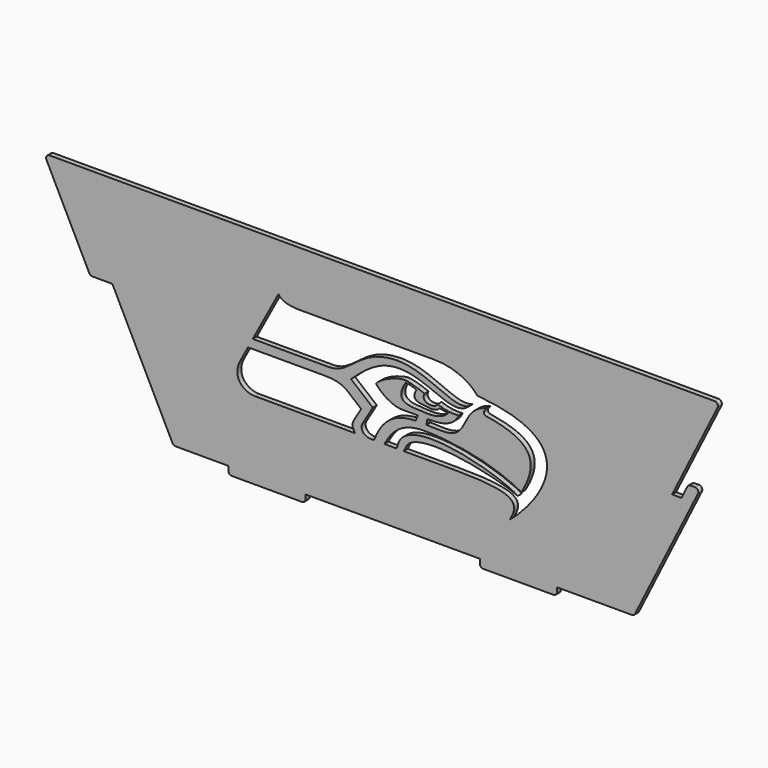
from build123d import *

# Parameters (mm, degrees)
F1_DEPTH = 4.7625
F3_DEPTH = 4.7635


with BuildPart() as f1:
    # F0 (on Front) → F1 (new body)
    with BuildSketch(Plane.XZ):
        with BuildLine():
            Line((304.8471037094, 203.7780743591), (-309.9778465366, 203.7780743591))
            Line((-309.9778465366, 203.7780743591), (-325.0692571728, 203.7780743591))
            ThreePointArc((-325.0692571728, 203.7780743591), (-327.7691254871, 202.2738035667), (-327.9106737709, 199.1863963025))
            Line((-327.9106737709, 199.1863963025), (-287.3259657756, 117.7860651637))
            ThreePointArc((-287.3259657756, 117.7860651637), (-286.1552783851, 116.502874906), (-284.4845491775, 116.0277432204))
            Line((-284.4845491775, 116.0277432204), (-265.4942987936, 116.0277432204))
            Line((-265.4942987936, 116.0277432204), (-208.521666982, 1.7583219434))
            ThreePointArc((-208.521666982, 1.7583219434), (-207.3509795915, 0.4751316856), (-205.6802503839, 0))
            Line((-205.6802503839, 0), (-155.575, 0))
            Line((-155.575, 0), (-155.575, -4.191))
            ThreePointArc((-155.575, -4.191), (-154.6450640303, -6.4360640303), (-152.4, -7.366))
            Line((-152.4, -7.366), (-85.725, -7.366))
            ThreePointArc((-85.725, -7.366), (-83.4799359697, -6.4360640303), (-82.55, -4.191))
            Line((-82.55, -4.191), (-82.55, 0))
            Line((-82.55, 0), (82.55, 0))
            Line((82.55, 0), (82.55, -4.191))
            ThreePointArc((82.55, -4.191), (83.4799359697, -6.4360640303), (85.725, -7.366))
            Line((85.725, -7.366), (152.4, -7.366))
            ThreePointArc((152.4, -7.366), (154.6450640303, -6.4360640303), (155.575, -4.191))
            Line((155.575, -4.191), (155.575, 0))
            Line((155.575, 0), (226.6352503839, 0))
            ThreePointArc((226.6352503839, 0), (228.3059795915, 0.4751316856), (229.476666982, 1.7583219434))
            Line((229.476666982, 1.7583219434), (289.1203551674, 121.3850534994))
            ThreePointArc((289.1203551674, 121.3850534994), (288.9788068837, 124.4724607637), (286.2789385693, 125.9767315561))
            Line((286.2789385693, 125.9767315561), (282.0216431033, 125.9767315561))
            ThreePointArc((282.0216431033, 125.9767315561), (280.3509138957, 125.5015998704), (279.1802265053, 124.2184096127))
            Line((279.1802265053, 124.2184096127), (273.5135142788, 112.8527432204))
            Line((273.5135142788, 112.8527432204), (264.6441487246, 112.8527432204))
            Line((264.6441487246, 112.8527432204), (307.6885203074, 199.1863963025))
            ThreePointArc((307.6885203074, 199.1863963025), (307.5469720237, 202.2738035667), (304.8471037094, 203.7780743591))
        make_face()
    extrude(amount=-F1_DEPTH)

    # F2 (on face) → F3 (cut, through all)
    with BuildSketch(Plane.XZ):
        with BuildLine():
            add(Edge.make_bspline(
                [(-108.0855709555, 158.8200743591), (-104.9123463275, 152.4905528223), (-92.8046389769, 151.9620743591), (-89.1326591372, 151.9620743591)],
                knots=[0, 0, 0, 0, 20.1555210895, 20.1555210895, 20.1555210895, 20.1555210895], degree=3))
            Line((-108.0855709555, 158.8200743591), (-132.5024012116, 113.3540743591))
            Line((-132.5024012116, 113.3540743591), (-60.2126787959, 113.3540743591))
            add(Edge.make_bspline(
                [(-60.2126787959, 113.3540743591), (-39.1802881973, 113.3540743591), (-32.2392965277, 139.1934752464), (3.4948316792, 139.8413479328)],
                knots=[0, 0, 0, 0, 68.994366091, 68.994366091, 68.994366091, 68.994366091], degree=3))
            add(Edge.make_bspline(
                [(3.4948316792, 139.8413479328), (33.620741922, 140.3875415964), (57.5292114558, 116.1221712828), (72.603527868, 124.0668594837)],
                knots=[0, 0, 0, 0, 70.8861507965, 70.8861507965, 70.8861507965, 70.8861507965], degree=3))
            add(Edge.make_bspline(
                [(72.603527868, 124.0668594837), (57.3887829127, 108.9602857828), (35.1666625979, 133.7167322636), (6.5191294456, 133.8571608067)],
                knots=[0, 0, 0, 0, 66.8056712775, 66.8056712775, 66.8056712775, 66.8056712775], degree=3))
            add(Edge.make_bspline(
                [(6.5191294456, 133.8571608067), (-10.7343354961, 133.9417362894), (-23.3095789241, 125.1955926418), (-39.4589209842, 110.169686377)],
                knots=[0, 0, 0, 0, 51.721152019, 51.721152019, 51.721152019, 51.721152019], degree=3))
            Line((-39.4589209842, 110.169686377), (-18.8014073711, 93.0641664272))
            Line((-18.8014073711, 93.0641664272), (-28.5283795675, 76.7167973694))
            add(Edge.make_bspline(
                [(-28.5283795675, 76.7167973694), (-31.1035539324, 72.3889011976), (-28.2070931256, 66.294), (-19.8544518154, 66.294)],
                knots=[0, 0, 0, 0, 13.5599309604, 13.5599309604, 13.5599309604, 13.5599309604], degree=3))
            Line((-19.8544518154, 66.294), (-17.6944385452, 66.294))
            Line((-17.6944385452, 66.294), (-15.5441686511, 71.12))
            add(Edge.make_bspline(
                [(21.8052406029, 95.3664587708), (7.467065883, 94.8295469973), (-6.8637521331, 90.6020614063), (-15.5441686511, 71.12)],
                knots=[43.7475476307, 43.7475476307, 43.7475476307, 43.7475476307, 82.7254389845, 82.7254389845, 82.7254389845, 82.7254389845], degree=3))
            Line((21.8052406029, 95.3664587708), (23.9405263848, 100.4171879244))
            Line((23.9405263848, 100.4171879244), (9.3578106412, 100.4171879244))
            add(Edge.make_bspline(
                [(-15.7739197216, 113.8468384743), (-9.2178139216, 106.1980500817), (0.431748606, 100.4171879244), (9.3578106412, 100.4171879244)],
                knots=[0, 0, 0, 0, 28.4949010337, 28.4949010337, 28.4949010337, 28.4949010337], degree=3))
            add(Edge.make_bspline(
                [(13.4090365761, 125.7664517022), (6.1268161537, 127.0878911018), (-12.3137527457, 119.4923743606), (-15.7739197216, 113.8468384743)],
                knots=[0, 0, 0, 0, 31.5233582883, 31.5233582883, 31.5233582883, 31.5233582883], degree=3))
            add(Edge.make_bspline(
                [(13.4090365761, 125.7664517022), (17.0461437806, 125.1064583922), (20.456541102, 124.1535529113), (23.7161297893, 123.0590063051)],
                knots=[0, 0, 0, 0, 9.7414046888, 9.7414046888, 9.7414046888, 9.7414046888], degree=3))
            add(Edge.make_bspline(
                [(23.7161297893, 123.0590063051), (25.9461937878, 122.3101667382), (28.1056690745, 121.4950294779), (30.2188615937, 120.6620362251)],
                knots=[9.7414046888, 9.7414046888, 9.7414046888, 9.7414046888, 16.4060357128, 16.4060357128, 16.4060357128, 16.4060357128], degree=3))
            add(Edge.make_bspline(
                [(30.2188615937, 120.6620362251), (34.4613134246, 118.989716397), (38.5172239418, 117.2454285237), (42.5832667432, 115.8211427133)],
                knots=[16.4060357128, 16.4060357128, 16.4060357128, 16.4060357128, 29.785969549, 29.785969549, 29.785969549, 29.785969549], degree=3))
            add(Edge.make_bspline(
                [(42.5832667432, 115.8211427133), (43.6102126796, 115.4614159232), (44.6378049525, 115.1221020021), (45.6692122023, 114.8095160445)],
                knots=[29.785969549, 29.785969549, 29.785969549, 29.785969549, 33.1652917436, 33.1652917436, 33.1652917436, 33.1652917436], degree=3))
            add(Edge.make_bspline(
                [(45.6692122023, 114.8095160445), (48.3287241294, 114.0035045657), (51.0136010899, 113.3752020751), (53.778166648, 113.0328753327)],
                knots=[33.1652917436, 33.1652917436, 33.1652917436, 33.1652917436, 41.8789668545, 41.8789668545, 41.8789668545, 41.8789668545], degree=3))
            add(Edge.make_bspline(
                [(53.778166648, 113.0328753327), (56.6101394852, 112.6822017765), (59.5257343252, 112.6316196452), (62.5833460553, 112.9975098393)],
                knots=[41.8789668545, 41.8789668545, 41.8789668545, 41.8789668545, 50.8051039667, 50.8051039667, 50.8051039667, 50.8051039667], degree=3))
            add(Edge.make_bspline(
                [(62.5833460553, 112.9975098393), (57.5499871238, 101.6970577857), (44.895685374, 100.4171879244), (35.6732808673, 100.4171879244)],
                knots=[0, 0, 0, 0, 29.7054895248, 29.7054895248, 29.7054895248, 29.7054895248], degree=3))
            Line((35.6732808673, 100.4171879244), (32.955760204, 100.4171879244))
            Line((32.955760204, 100.4171879244), (31.936584741, 95.2798231627))
            add(Edge.make_bspline(
                [(62.1327087283, 99.5770022273), (55.7191114325, 93.5406797473), (44.3494086047, 94.7811794741), (31.936584741, 95.2798231627)],
                knots=[0, 0, 0, 0, 34.4997978654, 34.4997978654, 34.4997978654, 34.4997978654], degree=3))
            add(Edge.make_bspline(
                [(89.5263329148, 127.8310716152), (69.5112124085, 122.403241694), (71.6838326954, 108.5662888403), (62.1327087283, 99.5770022273)],
                knots=[0, 0, 0, 0, 39.3535650615, 39.3535650615, 39.3535650615, 39.3535650615], degree=3))
            add(Edge.make_bspline(
                [(88.5086134076, 120.820119977), (86.8319925342, 121.0770893363), (84.3538343906, 123.8052621484), (89.5263329148, 127.8310716152)],
                knots=[0, 0, 0, 0, 7.0844333485, 7.0844333485, 7.0844333485, 7.0844333485], degree=3))
            add(Edge.make_bspline(
                [(121.9802498817, 68.2379975915), (138.7160643935, 97.1864387393), (133.5143968463, 113.9222532511), (88.5086134076, 120.820119977)],
                knots=[0, 0, 0, 0, 62.3316135105, 62.3316135105, 62.3316135105, 62.3316135105], degree=3))
            add(Edge.make_bspline(
                [(47.0553375781, 88.7687131763), (73.0637013912, 86.6201967001), (100.202858448, 80.1746398211), (121.9802498817, 68.2379975915)],
                knots=[0, 0, 0, 0, 77.6868892809, 77.6868892809, 77.6868892809, 77.6868892809], degree=3))
            add(Edge.make_bspline(
                [(-4.9613900483, 71.12), (7.5904717669, 91.8218642473), (26.8748909697, 90.4357931335), (47.0553375781, 88.7687131763)],
                knots=[0, 0, 0, 0, 54.9292001556, 54.9292001556, 54.9292001556, 54.9292001556], degree=3))
            Line((-4.9613900483, 71.12), (-7.8874688012, 66.294))
            Line((-7.8874688012, 66.294), (3.7596509099, 66.294))
            Line((3.7596509099, 66.294), (5.3652498768, 71.12))
            add(Edge.make_bspline(
                [(118.5127422214, 64.0348792076), (101.5507727861, 75.9082660079), (15.1123561065, 100.4171879244), (5.3652498768, 71.12)],
                knots=[0, 0, 0, 0, 113.3691049647, 113.3691049647, 113.3691049647, 113.3691049647], degree=3))
            add(Edge.make_bspline(
                [(12.9629354924, 71.12), (22.3948843777, 89.7157178473), (96.2360203266, 73.8728269935), (118.5127422214, 64.0348792076)],
                knots=[0, 0, 0, 0, 105.7873368469, 105.7873368469, 105.7873368469, 105.7873368469], degree=3))
            Line((12.9629354924, 71.12), (10.5151361821, 66.294))
            Line((10.5151361821, 66.294), (56.5995481846, 66.294))
            add(Edge.make_bspline(
                [(56.5995481846, 66.294), (110.5179414153, 66.294), (122.5627437234, 60.7635602355), (110.8795709555, 41.91)],
                knots=[0, 0, 0, 0, 59.5054646903, 59.5054646903, 59.5054646903, 59.5054646903], degree=3))
            add(Edge.make_bspline(
                [(80.1455709555, 135.1980743591), (200.1843783476, 125.0355941836), (122.1671178937, 50.3128953278), (110.8795709555, 41.91)],
                knots=[0, 0, 0, 0, 98.2203826791, 98.2203826791, 98.2203826791, 98.2203826791], degree=3))
            add(Edge.make_bspline(
                [(39.4882895052, 151.9620743591), (56.6352656532, 151.9620743591), (72.1557098843, 145.339655656), (80.1455709555, 135.1980743591)],
                knots=[0, 0, 0, 0, 43.9777924744, 43.9777924744, 43.9777924744, 43.9777924744], degree=3))
            Line((39.4882895052, 151.9620743591), (-89.1326591372, 151.9620743591))
        make_face()
        with BuildLine():
            add(Edge.make_bspline(
                [(12.3068088502, 124.0342240695), (1.1161545615, 105.8044293233), (14.6102500618, 105.6872327259), (25.9561562797, 105.1848872923)],
                knots=[0.7102763311, 0.7102763311, 0.7102763311, 0.7102763311, 23.8266655087, 23.8266655087, 23.8266655087, 23.8266655087], degree=3))
            add(Edge.make_bspline(
                [(25.9561562797, 105.1848872923), (27.0228511647, 105.1376588653), (28.0705582522, 105.0870261162), (29.0769792648, 105.0176173449)],
                knots=[23.8266655087, 23.8266655087, 23.8266655087, 23.8266655087, 25.999972217, 25.999972217, 25.999972217, 25.999972217], degree=3))
            add(Edge.make_bspline(
                [(29.0769792648, 105.0176173449), (30.4571273904, 104.9224341319), (32.0740966925, 104.8272509189), (33.8305222972, 104.8266072203)],
                knots=[0, 0, 0, 0, 5.6185155122, 5.6185155122, 5.6185155122, 5.6185155122], degree=3))
            add(Edge.make_bspline(
                [(33.8305222972, 104.8266072203), (39.8153318399, 104.8244138946), (47.419262347, 105.9198468996), (52.7905111522, 111.8529362833)],
                knots=[5.6185155122, 5.6185155122, 5.6185155122, 5.6185155122, 24.7629331084, 24.7629331084, 24.7629331084, 24.7629331084], degree=3))
            add(Edge.make_bspline(
                [(44.736277312, 113.2977232337), (46.8287324835, 112.3291605312), (49.5715110012, 112.1103200926), (52.7905111522, 111.8529362833)],
                knots=[0, 0, 0, 0, 8.1827924381, 8.1827924381, 8.1827924381, 8.1827924381], degree=3))
            add(Edge.make_bspline(
                [(31.936584741, 110.4435324669), (36.1832783119, 109.8596122357), (41.7581351236, 109.4985063713), (44.736277312, 113.2977232337)],
                knots=[0, 0, 0, 0, 12.8997037507, 12.8997037507, 12.8997037507, 12.8997037507], degree=3))
            add(Edge.make_bspline(
                [(22.5016381862, 121.1884725319), (16.3800276877, 110.9197529051), (26.3885025587, 111.2063935908), (31.936584741, 110.4435324669)],
                knots=[0.8157155355, 0.8157155355, 0.8157155355, 0.8157155355, 15.0574254033, 15.0574254033, 15.0574254033, 15.0574254033], degree=3))
            add(Edge.make_bspline(
                [(12.3068088502, 124.0342240695), (16.6386780488, 123.5824419574), (20.4999645308, 122.2686762918), (22.5016381862, 121.1884725319)],
                knots=[0, 0, 0, 0, 10.5845570056, 10.5845570056, 10.5845570056, 10.5845570056], degree=3))
        make_face()
        with BuildLine():
            add(Edge.make_bspline(
                [(30.2188615937, 120.6620362251), (34.4613134246, 118.989716397), (38.5172239418, 117.2454285237), (42.5832667432, 115.8211427133)],
                knots=[16.4060357128, 16.4060357128, 16.4060357128, 16.4060357128, 29.785969549, 29.785969549, 29.785969549, 29.785969549], degree=3))
            add(Edge.make_bspline(
                [(30.2188615937, 120.6620362251), (25.5965165799, 112.7740041532), (39.6847280117, 110.4019199935), (42.5832667432, 115.8211427133)],
                knots=[0, 0, 0, 0, 13.278281692, 13.278281692, 13.278281692, 13.278281692], degree=3))
        make_face()
        with BuildLine():
            add(Edge.make_bspline(
                [(-144.4075709555, 91.1857403905), (-152.2815709555, 76.5237519078), (-141.7369842529, 66.294), (-130.2270442247, 66.294)],
                knots=[0, 0, 0, 0, 28.6476190639, 28.6476190639, 28.6476190639, 28.6476190639], degree=3))
            Line((-130.2270442247, 66.294), (-35.6024518154, 66.294))
            add(Edge.make_bspline(
                [(-35.6024518154, 78.7363988543), (-38.9614162178, 73.0912474517), (-38.7686877988, 71.3825975361), (-35.6024518154, 66.294)],
                knots=[0, 0, 0, 0, 12.4423988543, 12.4423988543, 12.4423988543, 12.4423988543], degree=3))
            Line((-35.6024518154, 78.7363988543), (-29.8666387812, 88.3761357246))
            Line((-29.8666387812, 88.3761357246), (-42.6043234766, 98.9236161113))
            add(Edge.make_bspline(
                [(-63.8894603974, 104.902), (-54.1243873339, 104.902), (-47.3529842716, 102.8557598091), (-42.6043234766, 98.9236161113)],
                knots=[0, 0, 0, 0, 22.1087794249, 22.1087794249, 22.1087794249, 22.1087794249], degree=3))
            Line((-63.8894603974, 104.902), (-137.0414603974, 104.902))
            Line((-137.0414603974, 104.902), (-144.4075709555, 91.1857403905))
        make_face()
    extrude(amount=-F3_DEPTH, mode=Mode.SUBTRACT)


solid = f1.part
